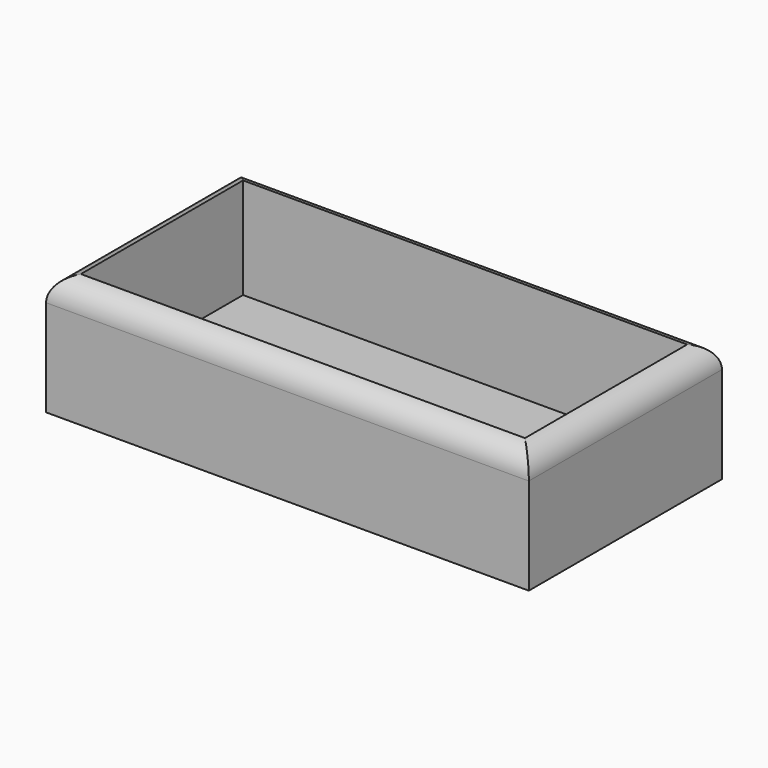
from build123d import *

# Parameters (mm, degrees)
F0_W        = 100
F0_H        = 50
F1_DEPTH    = 25
F2_T        = -4
F3_T1_DEPTH = 75
F3_T3_DEPTH = 125


# Not quite as in the source:
# - a fillet or chamfer that OpenCascade refuses, or shapes differently, is made with other operations: its cross-section is extruded or revolved along the edge and cut away or added


with BuildPart() as f1:
    # F0 (on Top) → F1 (new body)
    with BuildSketch(Plane.XY):
        with Locations((-4.7528631985, -11.9245312498)):
            Rectangle(F0_W, F0_H)
    extrude(amount=F1_DEPTH)

    # F2
    f2_openings = [f1.faces().sort_by_distance(p)[0] for p in [
        (-4.752863, -11.924531, 25),
    ]]
    offset(amount=F2_T, openings=f2_openings)

    # F3: fillet of radius 5 on 4 edges, made by hand

    # F3_s2 → F3_t1 (cut)
    with BuildSketch(Plane.XZ.offset(-25.5754687502)):
        with BuildLine():
            ThreePointArc((-54.7528631985, 20), (-53.2883971045, 23.5355339059), (-49.7528631985, 25))
            Line((-49.7528631985, 25), (-54.7528631985, 25))
            Line((-54.7528631985, 25), (-54.7528631985, 20))
        make_face()
        with BuildLine():
            ThreePointArc((45.2471368015, 20), (43.7826707074, 23.5355339059), (40.2471368015, 25))
            Line((40.2471368015, 25), (45.2471368015, 25))
            Line((45.2471368015, 25), (45.2471368015, 20))
        make_face()
    extrude(amount=F3_T1_DEPTH, mode=Mode.SUBTRACT)

    # F3_s4 → F3_t3 (cut)
    with BuildSketch(Plane.YZ.offset(-67.2528631985)):
        with BuildLine():
            ThreePointArc((13.0754687502, 20), (11.6110026561, 23.5355339059), (8.0754687502, 25))
            Line((8.0754687502, 25), (13.0754687502, 25))
            Line((13.0754687502, 25), (13.0754687502, 20))
        make_face()
        with BuildLine():
            ThreePointArc((-36.9245312498, 20), (-35.4600651557, 23.5355339059), (-31.9245312498, 25))
            Line((-31.9245312498, 25), (-36.9245312498, 25))
            Line((-36.9245312498, 25), (-36.9245312498, 20))
        make_face()
    extrude(amount=F3_T3_DEPTH, mode=Mode.SUBTRACT)


solid = f1.part
